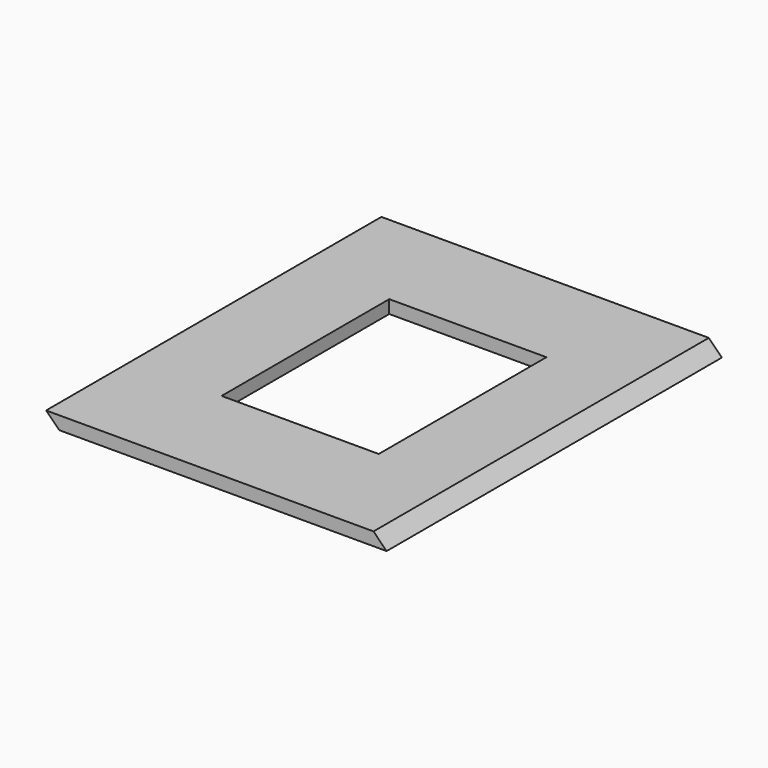
from build123d import *

# Parameters (mm, degrees)
F0_W     = 82.55
F0_H     = 101.6
F1_DEPTH = 3.175
F2_SIZE  = 3.17499
F3_W     = 38.1
F3_H     = 50.8
F4_DEPTH = 3.175
F5_SIZE  = 3.17499


# Not quite as in the source:
# - a fillet or chamfer is up to 0.001 mm smaller than in the source, because OpenCascade refuses the exact size


with BuildPart() as f1:
    # F0 (on Top) → F1 (new body)
    with BuildSketch(Plane.XY):
        Rectangle(F0_W, F0_H)
    extrude(amount=F1_DEPTH)

    # F2 (size 3.175 in the source; OpenCascade refuses exactly that, so slightly less here)
    f2_edges = [f1.edges().sort_by_distance(p)[0] for p in [
        (-41.275, 0, 0),
    ]]
    chamfer(f2_edges, length=F2_SIZE)

    # F3 (on face) → F4 (cut)
    with BuildSketch(Plane(origin=(0, 0, 0), x_dir=(1, 0, 0), z_dir=(0, 0, -1))):
        Rectangle(F3_W, F3_H)
    extrude(amount=-F4_DEPTH, mode=Mode.SUBTRACT)

    # F5 (size 3.175 in the source; OpenCascade refuses exactly that, so slightly less here)
    f5_edges = [f1.edges().sort_by_distance(p)[0] for p in [
        (41.275, 0, 3.175),
    ]]
    chamfer(f5_edges, length=F5_SIZE)


solid = f1.part
